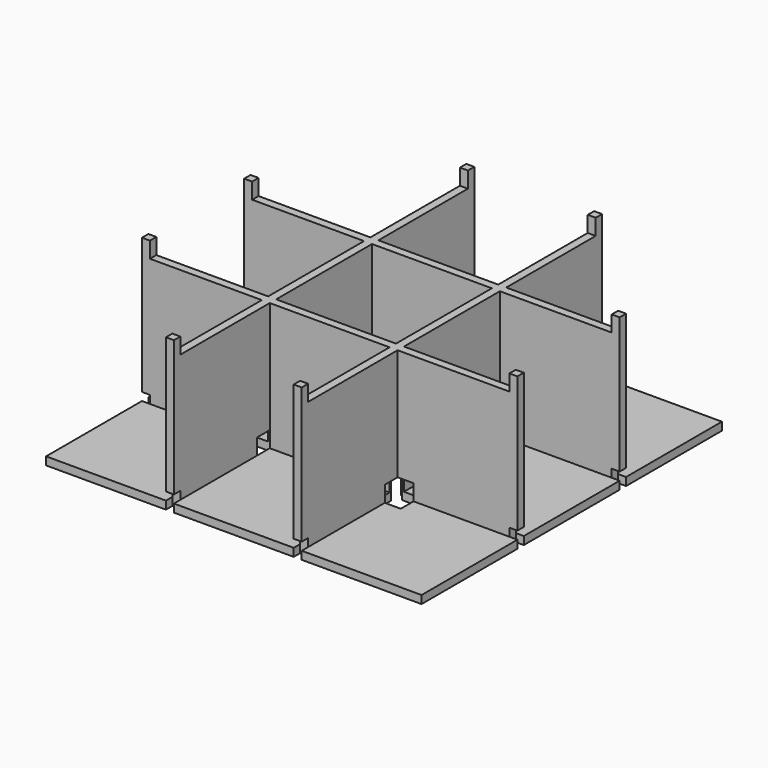
from build123d import *

# Parameters (mm, degrees)
F0_W          = 1
F0_H          = 15
F0_W_2        = 15
F0_H_2        = 1
F1_DEPTH      = 1
F2_DEPTH      = 16
F3_W          = 2
F3_H          = 3
F3_W_2        = 3
F3_H_2        = 2
F4_DEPTH      = 3
F5_W          = 1
F5_H          = 1
F6_DEPTH      = 25
F7_DEPTH      = 2
F7_DEPTH_BACK = 15


with BuildPart() as f1:
    # F0 (on Top) → F1 (new body)
    with BuildSketch(Plane.XY):
        with Locations((8, 0)):
            Rectangle(F0_W, F0_H)
        with Locations((-16, -8)):
            Rectangle(F0_W_2, F0_H_2)
        with Locations((-16, 0)):
            Rectangle(F0_W_2, F0_H)
        with Locations((8, -16)):
            Rectangle(F0_W, F0_H)
        with Locations((0, -16)):
            Rectangle(F0_W_2, F0_H)
        with Locations((-8, -16)):
            Rectangle(F0_W, F0_H)
        with Locations((16, -16)):
            Rectangle(F0_W_2, F0_H)
        with Locations((-16, -16)):
            Rectangle(F0_W_2, F0_H)
        with Locations((16, 0)):
            Rectangle(F0_W_2, F0_H)
        with Locations((16, -8)):
            Rectangle(F0_W_2, F0_H_2)
        with Locations((0, -8)):
            Rectangle(F0_W_2, F0_H_2)
        with Locations((-8, 0)):
            Rectangle(F0_W, F0_H)
        Rectangle(F0_W_2, F0_H)
        with Locations((8, -8)):
            Rectangle(F0_W, F0_H_2)
        with Locations((-8, -8)):
            Rectangle(F0_W, F0_H_2)
        with Locations((-8, 8)):
            Rectangle(F0_W, F0_H_2)
        with Locations((-16, 8)):
            Rectangle(F0_W_2, F0_H_2)
        with Locations((8, 16)):
            Rectangle(F0_W, F0_H)
        with Locations((0, 16)):
            Rectangle(F0_W_2, F0_H)
        with Locations((-8, 16)):
            Rectangle(F0_W, F0_H)
        with Locations((16, 16)):
            Rectangle(F0_W_2, F0_H)
        with Locations((16, 8)):
            Rectangle(F0_W_2, F0_H_2)
        with Locations((-16, 16)):
            Rectangle(F0_W_2, F0_H)
        with Locations((8, 8)):
            Rectangle(F0_W, F0_H_2)
        with Locations((0, 8)):
            Rectangle(F0_W_2, F0_H_2)
    extrude(amount=-F1_DEPTH)

    # F0 (on Top) → F2 (join)
    with BuildSketch(Plane.XY):
        with Locations((-8, -8)):
            Rectangle(F0_W, F0_H_2)
        with Locations((8, -8)):
            Rectangle(F0_W, F0_H_2)
        with Locations((-8, 8)):
            Rectangle(F0_W, F0_H_2)
        with Locations((8, 8)):
            Rectangle(F0_W, F0_H_2)
        with Locations((16, 8)):
            Rectangle(F0_W_2, F0_H_2)
        with Locations((8, 16)):
            Rectangle(F0_W, F0_H)
        with Locations((-8, 16)):
            Rectangle(F0_W, F0_H)
        with Locations((0, 8)):
            Rectangle(F0_W_2, F0_H_2)
        with Locations((-16, 8)):
            Rectangle(F0_W_2, F0_H_2)
        with Locations((-8, 0)):
            Rectangle(F0_W, F0_H)
        with Locations((-16, -8)):
            Rectangle(F0_W_2, F0_H_2)
        with Locations((0, -8)):
            Rectangle(F0_W_2, F0_H_2)
        with Locations((16, -8)):
            Rectangle(F0_W_2, F0_H_2)
        with Locations((8, -16)):
            Rectangle(F0_W, F0_H)
        with Locations((-8, -16)):
            Rectangle(F0_W, F0_H)
        with Locations((8, 0)):
            Rectangle(F0_W, F0_H)
    extrude(amount=F2_DEPTH)

    # F3 (on face) → F4 (cut)
    with BuildSketch(Plane(origin=(0, 0, -1), x_dir=(1, 0, 0), z_dir=(0, 0, -1))):
        with BuildLine():
            Line((-7.5, 8.25), (-7.5, 7.5))
            Line((-7.5, 7.5), (-6.75, 7.5))
            ThreePointArc((-6.75, 7.5), (-6.9696699141, 8.0303300859), (-7.5, 8.25))
        make_face()
        with BuildLine():
            Line((-6.75, 7.5), (-7.5, 7.5))
            Line((-7.5, 7.5), (-7.5, 6.75))
            ThreePointArc((-7.5, 6.75), (-6.9696699141, 6.9696699141), (-6.75, 7.5))
        make_face()
        with BuildLine():
            Line((-7.5, 6.75), (-7.5, 7.5))
            Line((-7.5, 7.5), (-8.25, 7.5))
            ThreePointArc((-8.25, 7.5), (-8.0303300859, 6.9696699141), (-7.5, 6.75))
        make_face()
        with BuildLine():
            Line((-8.25, 7.5), (-7.5, 7.5))
            Line((-7.5, 7.5), (-7.5, 8.25))
            ThreePointArc((-7.5, 8.25), (-8.0303300859, 8.0303300859), (-8.25, 7.5))
        make_face()
        with BuildLine():
            Line((-1, 7.5), (-6.75, 7.5))
            ThreePointArc((-6.75, 7.5), (-6.9696699141, 6.9696699141), (-7.5, 6.75))
            Line((-7.5, 6.75), (-7.5, 1))
            Line((-7.5, 1), (-7.5, -1))
            Line((-7.5, -1), (-7.5, -6.75))
            ThreePointArc((-7.5, -6.75), (-6.9696699141, -6.9696699141), (-6.75, -7.5))
            Line((-6.75, -7.5), (-1, -7.5))
            Line((-1, -7.5), (1, -7.5))
            Line((1, -7.5), (6.75, -7.5))
            ThreePointArc((6.75, -7.5), (6.9696699141, -6.9696699141), (7.5, -6.75))
            Line((7.5, -6.75), (7.5, -1))
            Line((7.5, -1), (7.5, 1))
            Line((7.5, 1), (7.5, 6.75))
            ThreePointArc((7.5, 6.75), (6.9696699141, 6.9696699141), (6.75, 7.5))
            Line((6.75, 7.5), (1, 7.5))
            Line((1, 7.5), (-1, 7.5))
        make_face()
        with BuildLine():
            Line((-10.5, 7.5), (-8.25, 7.5))
            ThreePointArc((-8.25, 7.5), (-8.0303300859, 8.0303300859), (-7.5, 8.25))
            Line((-7.5, 8.25), (-7.5, 10.5))
            Line((-7.5, 10.5), (-10.5, 10.5))
            Line((-10.5, 10.5), (-10.5, 7.5))
        make_face()
        with Locations((0, 9)):
            Rectangle(F3_W, F3_H)
        with Locations((-9, 0)):
            Rectangle(F3_W_2, F3_H_2)
        with BuildLine():
            ThreePointArc((7.5, 8.25), (6.9696699141, 8.0303300859), (6.75, 7.5))
            Line((6.75, 7.5), (7.5, 7.5))
            Line((7.5, 7.5), (7.5, 8.25))
        make_face()
        with BuildLine():
            Line((7.5, 7.5), (6.75, 7.5))
            ThreePointArc((6.75, 7.5), (6.9696699141, 6.9696699141), (7.5, 6.75))
            Line((7.5, 6.75), (7.5, 7.5))
        make_face()
        with BuildLine():
            ThreePointArc((-6.75, -7.5), (-6.9696699141, -6.9696699141), (-7.5, -6.75))
            Line((-7.5, -6.75), (-7.5, -7.5))
            Line((-7.5, -7.5), (-6.75, -7.5))
        make_face()
        with BuildLine():
            Line((-7.5, -7.5), (-7.5, -6.75))
            ThreePointArc((-7.5, -6.75), (-8.0303300859, -6.9696699141), (-8.25, -7.5))
            Line((-8.25, -7.5), (-7.5, -7.5))
        make_face()
        with BuildLine():
            Line((8.25, 7.5), (7.5, 7.5))
            Line((7.5, 7.5), (7.5, 6.75))
            ThreePointArc((7.5, 6.75), (8.0303300859, 6.9696699141), (8.25, 7.5))
        make_face()
        with BuildLine():
            Line((7.5, 8.25), (7.5, 7.5))
            Line((7.5, 7.5), (8.25, 7.5))
            ThreePointArc((8.25, 7.5), (8.0303300859, 8.0303300859), (7.5, 8.25))
        make_face()
        with BuildLine():
            Line((7.5, 10.5), (7.5, 8.25))
            ThreePointArc((7.5, 8.25), (8.0303300859, 8.0303300859), (8.25, 7.5))
            Line((8.25, 7.5), (10.5, 7.5))
            Line((10.5, 7.5), (10.5, 10.5))
            Line((10.5, 10.5), (7.5, 10.5))
        make_face()
        with BuildLine():
            Line((-7.5, -8.25), (-7.5, -7.5))
            Line((-7.5, -7.5), (-8.25, -7.5))
            ThreePointArc((-8.25, -7.5), (-8.0303300859, -8.0303300859), (-7.5, -8.25))
        make_face()
        with BuildLine():
            Line((-6.75, -7.5), (-7.5, -7.5))
            Line((-7.5, -7.5), (-7.5, -8.25))
            ThreePointArc((-7.5, -8.25), (-6.9696699141, -8.0303300859), (-6.75, -7.5))
        make_face()
        with BuildLine():
            ThreePointArc((-7.5, -8.25), (-8.0303300859, -8.0303300859), (-8.25, -7.5))
            Line((-8.25, -7.5), (-10.5, -7.5))
            Line((-10.5, -7.5), (-10.5, -10.5))
            Line((-10.5, -10.5), (-7.5, -10.5))
            Line((-7.5, -10.5), (-7.5, -8.25))
        make_face()
        with Locations((9, 0)):
            Rectangle(F3_W_2, F3_H_2)
        with Locations((0, -9)):
            Rectangle(F3_W, F3_H)
        with BuildLine():
            ThreePointArc((8.25, -7.5), (8.0303300859, -6.9696699141), (7.5, -6.75))
            Line((7.5, -6.75), (7.5, -7.5))
            Line((7.5, -7.5), (8.25, -7.5))
        make_face()
        with BuildLine():
            Line((7.5, -7.5), (7.5, -6.75))
            ThreePointArc((7.5, -6.75), (6.9696699141, -6.9696699141), (6.75, -7.5))
            Line((6.75, -7.5), (7.5, -7.5))
        make_face()
        with BuildLine():
            Line((7.5, -7.5), (6.75, -7.5))
            ThreePointArc((6.75, -7.5), (6.9696699141, -8.0303300859), (7.5, -8.25))
            Line((7.5, -8.25), (7.5, -7.5))
        make_face()
        with BuildLine():
            Line((8.25, -7.5), (7.5, -7.5))
            Line((7.5, -7.5), (7.5, -8.25))
            ThreePointArc((7.5, -8.25), (8.0303300859, -8.0303300859), (8.25, -7.5))
        make_face()
        with BuildLine():
            Line((10.5, -7.5), (8.25, -7.5))
            ThreePointArc((8.25, -7.5), (8.0303300859, -8.0303300859), (7.5, -8.25))
            Line((7.5, -8.25), (7.5, -10.5))
            Line((7.5, -10.5), (10.5, -10.5))
            Line((10.5, -10.5), (10.5, -7.5))
        make_face()
    extrude(amount=-F4_DEPTH, mode=Mode.SUBTRACT)

    # F5 (on face) → F6 (cut)
    with BuildSketch(Plane.XY.offset(16)):
        with Locations((-8, 23)):
            Rectangle(F5_W, F5_H)
        with Locations((-23, 8)):
            Rectangle(F5_W, F5_H)
        with Locations((8, 23)):
            Rectangle(F5_W, F5_H)
        with Locations((23, 8)):
            Rectangle(F5_W, F5_H)
        with Locations((23, -8)):
            Rectangle(F5_W, F5_H)
        with Locations((8, -23)):
            Rectangle(F5_W, F5_H)
        with Locations((-8, -23)):
            Rectangle(F5_W, F5_H)
        with Locations((-23, -8)):
            Rectangle(F5_W, F5_H)
    extrude(amount=-F6_DEPTH, mode=Mode.SUBTRACT)

    # F5 (on face) → F7 (join, two sides)
    with BuildSketch(Plane.XY.offset(16)) as f7_sk:
        with Locations((-8, 23)):
            Rectangle(F5_W, F5_H)
        with Locations((-23, 8)):
            Rectangle(F5_W, F5_H)
        with Locations((8, 23)):
            Rectangle(F5_W, F5_H)
        with Locations((23, 8)):
            Rectangle(F5_W, F5_H)
        with Locations((23, -8)):
            Rectangle(F5_W, F5_H)
        with Locations((8, -23)):
            Rectangle(F5_W, F5_H)
        with Locations((-8, -23)):
            Rectangle(F5_W, F5_H)
        with Locations((-23, -8)):
            Rectangle(F5_W, F5_H)
    extrude(amount=F7_DEPTH)
    extrude(f7_sk.sketch, amount=-F7_DEPTH_BACK)


solid = f1.part
